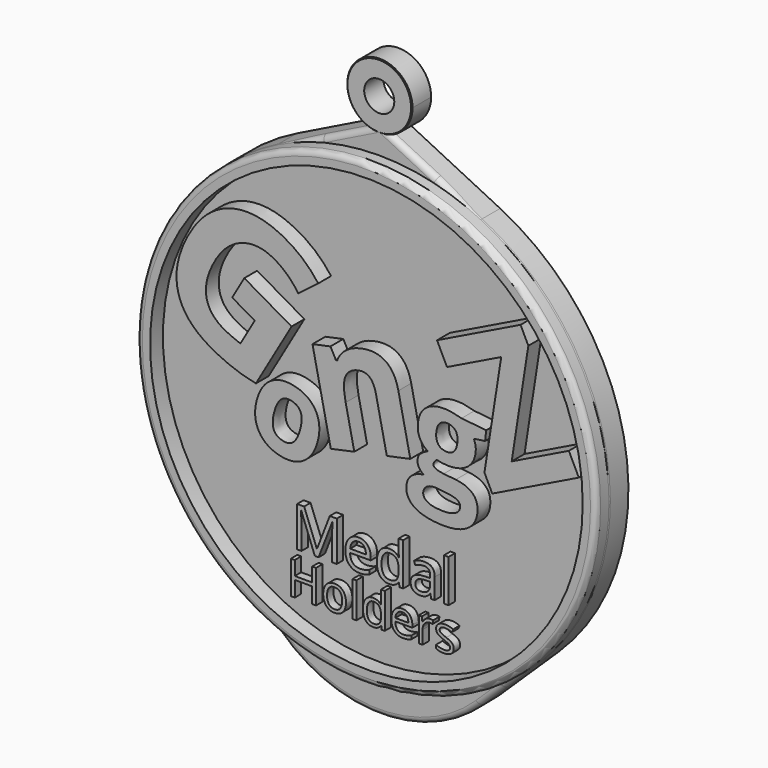
from build123d import *

# Parameters (mm, degrees)
F0_R            = 1.8741383758
F1_DEPTH        = 3
F2_R            = 28.6175176178
F2_R_2          = 26.9464151746
F3_DEPTH        = 2
F4_R            = 0.7
F5_SIZE         = 0.1
F6_TEXT_SIZE    = 23.9806039233
F7_DEPTH        = 2
F9_ANGLE        = 30
F11_TEXT_SIZE   = 14.8655256724
F12_DEPTH       = 2
F13_ANGLE       = 15
F15_TEXT_SIZE   = 20.0966183575
F16_DEPTH       = 2
F17_ANGLE       = -12
F19_TEXT_SIZE   = 16.1779575329
F20_DEPTH       = 2
F21_TEXT_SIZE   = 22.5806451613
F22_DEPTH       = 2
F24_ANGLE       = -26
F25_ANGLE       = 6
F27_TEXT_SIZE   = 6.9815643068
F27_TEXT_SIZE_2 = 5.7771491508
F28_DEPTH       = 1


# Not quite as in the source:
# - Text() gives the source's letters only with a copy of the font that has no kerning and outlines rounded to 1/6400 em; it was checked with that copy


with BuildPart() as f1:
    # F0 (on Front) → F1 (new body)
    with BuildSketch(Plane.XZ):
        with BuildLine():
            Line((12.5272742617, -27.7458937999), (19.9338672522, -20.5674681093))
            ThreePointArc((19.9338672522, -20.5674681093), (28.2946591849, 4.4488278984), (12.6603443468, 25.6923235438))
            Line((12.6603443468, 25.6923235438), (1.3355716254, 31.2728045018))
            ThreePointArc((1.3355716254, 31.2728045018), (0, 31.04717094), (-1.3355716254, 31.2728045018))
            Line((-1.3355716254, 31.2728045018), (-12.6603443468, 25.6923235438))
            ThreePointArc((-12.6603443468, 25.6923235438), (-28.2946591849, 4.4488278984), (-19.9338672522, -20.5674681093))
            Line((-19.9338672522, -20.5674681093), (-12.5272742617, -27.7458937999))
            ThreePointArc((-12.5272742617, -27.7458937999), (0, -32.8204383118), (12.5272742617, -27.7458937999))
        make_face()
        with BuildLine():
            ThreePointArc((-1.3355716254, 31.2728045018), (0, 31.04717094), (1.3355716254, 31.2728045018))
            ThreePointArc((1.3355716254, 31.2728045018), (3.3135180015, 32.7570057838), (4.0655788452, 35.1127497852))
            ThreePointArc((4.0655788452, 35.1127497852), (-2.3557440014, 38.4262677867), (-1.3355716254, 31.2728045018))
        make_face()
        with Locations((0, 35.1127497852)):
            Circle(F0_R, mode=Mode.SUBTRACT)
    extrude(amount=F1_DEPTH)

    # F2 (on face) → F3 (join)
    with BuildSketch(Plane.XZ.offset(3)):
        Circle(F2_R)
        Circle(F2_R_2, mode=Mode.SUBTRACT)
    extrude(amount=F3_DEPTH)

    # F4
    f4_edges = [f1.edges().sort_by_distance(p)[0] for p in [
        (0, -3, -32.820438),
        (16.230571, -3, -24.156681),
        (-16.230571, -3, -24.156681),
        (-28.617518, -5, 0),
    ]]
    fillet(f4_edges, radius=F4_R)

    # F5
    f5_edges = [f1.edges().sort_by_distance(p)[0] for p in [
        (0, -3, 39.178329),
    ]]
    chamfer(f5_edges, length=F5_SIZE)


with BuildPart() as f7:
    # F6 (on face) → F7 (new body)
    with BuildSketch(Plane.XZ.offset(3)):
        with Locations((-12.8745923461, -4.8888256371)):
            Text('G', F6_TEXT_SIZE, font='Open Sans', font_style=FontStyle.BOLD, text_align=(TextAlign.LEFT, TextAlign.BOTTOM))
    extrude(amount=F7_DEPTH)


with BuildPart() as f7_1:
    # F8: moved
    add(f7.part.moved(Location((-11.7, 0, 4.6))))


with BuildPart() as f7_2:
    # F9: moved
    add(f7_1.part.rotate(Axis((-15.9228400869, -4, 6.3020934725), (0, 1, 0)), F9_ANGLE))


with BuildPart() as f7_3:
    # F10: moved
    add(f7_2.part.moved(Location((-0.8, 0, 2.1))))


with BuildPart() as f12:
    # F11 (on face) → F12 (new body)
    with BuildSketch(Plane.XZ.offset(3)):
        with Locations((-3.721600584, -7.7860245308)):
            Text('o', F11_TEXT_SIZE, font='Open Sans', font_style=FontStyle.BOLD, text_align=(TextAlign.LEFT, TextAlign.BOTTOM))
    extrude(amount=F12_DEPTH)


with BuildPart() as f12_1:
    # F13: moved
    add(f12.part.rotate(Axis((2.5497930591, -4, -3.7142641396), (0, 1, 0)), F13_ANGLE))


with BuildPart() as f12_2:
    # F14: moved
    add(f12_1.part.moved(Location((-10.8, 0, 0.4))))


with BuildPart() as f16:
    # F15 (on face) → F16 (new body)
    with BuildSketch(Plane.XZ.offset(3)):
        with Locations((5.1382737488, -9.2035108604)):
            Text('n', F15_TEXT_SIZE, font='Open Sans', font_style=FontStyle.BOLD, text_align=(TextAlign.LEFT, TextAlign.BOTTOM))
    extrude(amount=F16_DEPTH)


with BuildPart() as f16_1:
    # F17: moved
    add(f16.part.rotate(Axis((13.8426215748, -4, -9.2035108604), (0, 1, 0)), F17_ANGLE))


with BuildPart() as f16_2:
    # F18: moved
    add(f16_1.part.moved(Location((-11.3, 0, 6.5))))


with BuildPart() as f20:
    # F19 (on face) → F20 (new body)
    with BuildSketch(Plane.XZ.offset(3)):
        with Locations((9.7386002408, -3.9152812426)):
            Text('g', F19_TEXT_SIZE, font='Open Sans', font_style=FontStyle.BOLD, text_align=(TextAlign.LEFT, TextAlign.BOTTOM))
    extrude(amount=F20_DEPTH)


with BuildPart() as f22:
    # F21 (on face) → F22 (new body)
    with BuildSketch(Plane.XZ.offset(3)):
        with Locations((8.7425441385, -8.206320768)):
            Text('Z', F21_TEXT_SIZE, font='Open Sans', font_style=FontStyle.BOLD, text_align=(TextAlign.LEFT, TextAlign.BOTTOM))
    extrude(amount=F22_DEPTH)


with BuildPart() as f22_1:
    # F23: moved
    add(f22.part.moved(Location((-0.9, 0, 9.4))))


with BuildPart() as f22_2:
    # F24: moved
    add(f22_1.part.rotate(Axis((20.1701651062, -4, 15.1090018126), (0, 1, 0)), F24_ANGLE))


with BuildPart() as f20_1:
    # F25: moved
    add(f20.part.rotate(Axis((9.7866285523, -4, -5.3536027795), (0, 1, 0)), F25_ANGLE))


with BuildPart() as f20_2:
    # F26: moved
    add(f20_1.part.moved(Location((-4.8, 0, 0.2))))


with BuildPart() as f28:
    # F27 (on face) → F28 (new body)
    with BuildSketch(Plane.XZ.offset(3)):
        with Locations((-10.114545345, -17.2517942266)):
            Text('Medal', F27_TEXT_SIZE, font='Open Sans', text_align=(TextAlign.LEFT, TextAlign.BOTTOM))
        with Locations((-10.7695003971, -22.6388778538)):
            Text('Holders', F27_TEXT_SIZE_2, font='Open Sans', text_align=(TextAlign.LEFT, TextAlign.BOTTOM))
    extrude(amount=F28_DEPTH)


solid = Compound([f1.part, f7_3.part, f12_2.part, f16_2.part, f22_2.part, f20_2.part, f28.part])
